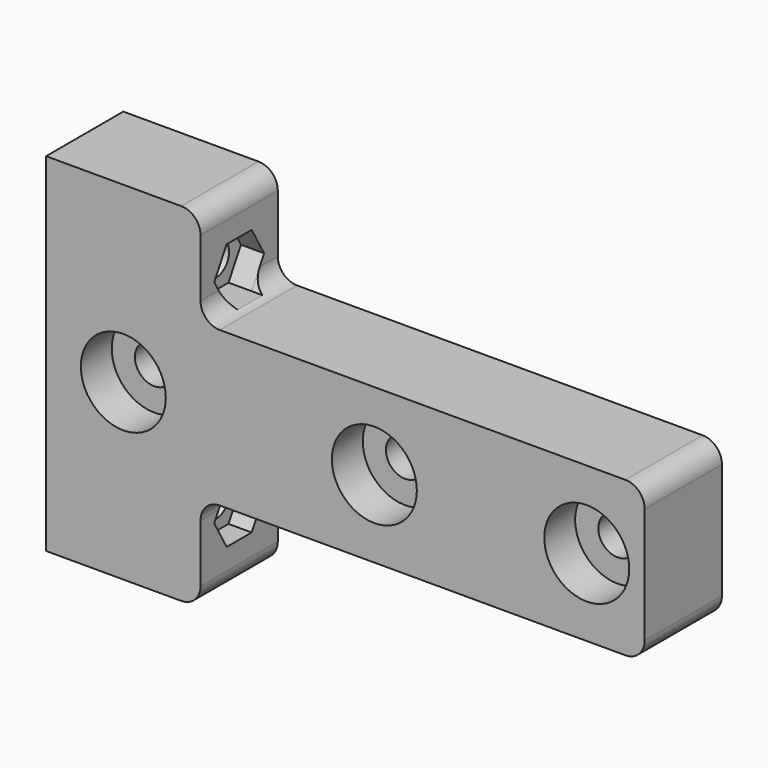
from build123d import *

# Parameters (mm, degrees)
F0_W          = 155
F0_H          = 40
F0_R          = 5
F1_DEPTH      = 25
F2_R          = 11
F3_DEPTH      = 10
F4_W          = 40
F4_H          = 25
F5_DEPTH      = 25
F6_R          = 4.25
F7_DEPTH      = 40
F9_DEPTH      = 6
F10_T4_DEPTH  = 25
F10_T10_DEPTH = 25
F10_T16_DEPTH = 25
F10_T23_DEPTH = 25
F10_T29_DEPTH = 25
F10_T35_DEPTH = 25
F10_T41_DEPTH = 25
F10_T47_DEPTH = 25
F10_T54_DEPTH = 25
F10_T60_DEPTH = 25
F10_T63_DEPTH = 50


# Not quite as in the source:
# - a fillet or chamfer that OpenCascade refuses, or shapes differently, is made with other operations: its cross-section is extruded or revolved along the edge and cut away or added


with BuildPart() as f1:
    # F0 (on Front) → F1 (new body)
    with BuildSketch(Plane.XZ):
        with Locations((-7.5, 0)):
            Rectangle(F0_W, F0_H)
        with Locations((-65, 0)):
            Circle(F0_R, mode=Mode.SUBTRACT)
        Circle(F0_R, mode=Mode.SUBTRACT)
        with Locations((55, 0)):
            Circle(F0_R, mode=Mode.SUBTRACT)
    extrude(amount=F1_DEPTH)

    # F2 (on face) → F3 (cut)
    with BuildSketch(Plane.XZ.offset(25)):
        with Locations((-65, 0)):
            Circle(F2_R)
        Circle(F2_R)
        with Locations((55, 0)):
            Circle(F2_R)
    extrude(amount=-F3_DEPTH, mode=Mode.SUBTRACT)

    # F4 (on face) → F5 (join)
    with BuildSketch(Plane(origin=(0, 0, 0), x_dir=(-1, 0, 0), z_dir=(0, 1, 0))):
        with Locations((65, 32.5)):
            Rectangle(F4_W, F4_H)
        with Locations((65, -32.5)):
            Rectangle(F4_W, F4_H)
    extrude(amount=-F5_DEPTH)

    # F6 (on face) → F7 (cut, through all)
    with BuildSketch(Plane(origin=(-85, 0, 0), x_dir=(0, -1, 0), z_dir=(-1, 0, 0))):
        with Locations((12.5, 27.5)):
            Circle(F6_R)
        with Locations((12.5, -27.5)):
            Circle(F6_R)
    extrude(amount=-F7_DEPTH, mode=Mode.SUBTRACT)

    # F8 (on face) → F9 (cut)
    with BuildSketch(Plane.YZ.offset(-45)):
        Polygon((-8.4585481157, 34.5), (-16.5414518843, 34.5), (-20.5829037687, 27.5), (-16.5414518843, 20.5), (-8.4585481157, 20.5), (-4.4170962313, 27.5), align=None)
        Polygon((-8.4585481157, -20.5), (-16.5414518843, -20.5), (-20.5829037687, -27.5), (-16.5414518843, -34.5), (-8.4585481157, -34.5), (-4.4170962313, -27.5), align=None)
    extrude(amount=-F9_DEPTH, mode=Mode.SUBTRACT)

    # F10: fillet of radius 5 on 6 edges, made by hand


with BuildPart() as f10_tool2:
    # F10_s3 → F10_t4 (new body)
    with BuildSketch(Plane.XZ):
        with BuildLine():
            ThreePointArc((-40, 20), (-43.5355339059, 21.4644660941), (-45, 25))
            Line((-45, 25), (-45, 20))
            Line((-45, 20), (-40, 20))
        make_face()
    extrude(amount=F10_T4_DEPTH)

    split(bisect_by=Plane.XY.offset(20.5), keep=Keep.BOTTOM)

    split(bisect_by=Plane(origin=(0, -15.2206714755, 8.7876587737), x_dir=(1, 0, 0), z_dir=(0, 0.8660254038, -0.5)), keep=Keep.TOP)


with BuildPart() as f1_1:
    add(f1.part)

    # F10_t1: union F10_tool2
    add(f10_tool2.part)


with BuildPart() as f10_tool8:
    # F10_s9 → F10_t10 (new body)
    with BuildSketch(Plane.XZ):
        with BuildLine():
            ThreePointArc((-40, 20), (-43.5355339059, 21.4644660941), (-45, 25))
            Line((-45, 25), (-45, 20))
            Line((-45, 20), (-40, 20))
        make_face()
    extrude(amount=F10_T10_DEPTH)

    split(bisect_by=Plane.XY.offset(20.5), keep=Keep.TOP)

    split(bisect_by=Plane(origin=(0, -15.2206714755, 8.7876587737), x_dir=(1, 0, 0), z_dir=(0, 0.8660254038, -0.5)), keep=Keep.TOP)


with BuildPart() as f1_2:
    add(f1_1.part)

    # F10_t7: union F10_tool8
    add(f10_tool8.part)


with BuildPart() as f10_tool14:
    # F10_s15 → F10_t16 (new body)
    with BuildSketch(Plane.XZ):
        with BuildLine():
            ThreePointArc((-40, 20), (-43.5355339059, 21.4644660941), (-45, 25))
            Line((-45, 25), (-45, 20))
            Line((-45, 20), (-40, 20))
        make_face()
    extrude(amount=F10_T16_DEPTH)

    split(bisect_by=Plane(origin=(0, -3.5293285245, -2.0376587737), x_dir=(1, 0, 0), z_dir=(0, 0.8660254038, 0.5)), keep=Keep.TOP)

    split(bisect_by=Plane.XY.offset(20.5), keep=Keep.BOTTOM)

    split(bisect_by=Plane(origin=(0, -15.2206714755, 8.7876587737), x_dir=(1, 0, 0), z_dir=(0, -0.8660254038, 0.5)), keep=Keep.TOP)


with BuildPart() as f1_3:
    add(f1_2.part)

    # F10_t13: union F10_tool14
    add(f10_tool14.part)


with BuildPart() as f10_tool21:
    # F10_s22 → F10_t23 (new body)
    with BuildSketch(Plane.XZ):
        with BuildLine():
            ThreePointArc((-40, 20), (-43.5355339059, 21.4644660941), (-45, 25))
            Line((-45, 25), (-45, 20))
            Line((-45, 20), (-40, 20))
        make_face()
    extrude(amount=F10_T23_DEPTH)

    split(bisect_by=Plane(origin=(0, -3.5293285245, -2.0376587737), x_dir=(1, 0, 0), z_dir=(0, -0.8660254038, -0.5)), keep=Keep.TOP)

    split(bisect_by=Plane.XY.offset(20.5), keep=Keep.BOTTOM)


with BuildPart() as f1_4:
    add(f1_3.part)

    # F10_t20: union F10_tool21
    add(f10_tool21.part)


with BuildPart() as f10_tool27:
    # F10_s28 → F10_t29 (new body)
    with BuildSketch(Plane.XZ):
        with BuildLine():
            ThreePointArc((-40, 20), (-43.5355339059, 21.4644660941), (-45, 25))
            Line((-45, 25), (-45, 20))
            Line((-45, 20), (-40, 20))
        make_face()
    extrude(amount=F10_T29_DEPTH)

    split(bisect_by=Plane(origin=(0, -3.5293285245, -2.0376587737), x_dir=(1, 0, 0), z_dir=(0, -0.8660254038, -0.5)), keep=Keep.TOP)

    split(bisect_by=Plane.XY.offset(20.5), keep=Keep.TOP)


with BuildPart() as f1_5:
    add(f1_4.part)

    # F10_t26: union F10_tool27
    add(f10_tool27.part)


with BuildPart() as f10_tool33:
    # F10_s34 → F10_t35 (new body)
    with BuildSketch(Plane.XZ):
        with BuildLine():
            ThreePointArc((-40, -20), (-43.5355339059, -21.4644660941), (-45, -25))
            Line((-45, -25), (-45, -20))
            Line((-45, -20), (-40, -20))
        make_face()
    extrude(amount=F10_T35_DEPTH)

    split(bisect_by=Plane.XY.offset(-20.5), keep=Keep.TOP)

    split(bisect_by=Plane(origin=(0, -15.2206714755, -8.7876587737), x_dir=(1, 0, 0), z_dir=(0, 0.8660254038, 0.5)), keep=Keep.TOP)


with BuildPart() as f1_6:
    add(f1_5.part)

    # F10_t32: union F10_tool33
    add(f10_tool33.part)


with BuildPart() as f10_tool39:
    # F10_s40 → F10_t41 (new body)
    with BuildSketch(Plane.XZ):
        with BuildLine():
            ThreePointArc((-40, -20), (-43.5355339059, -21.4644660941), (-45, -25))
            Line((-45, -25), (-45, -20))
            Line((-45, -20), (-40, -20))
        make_face()
    extrude(amount=F10_T41_DEPTH)

    split(bisect_by=Plane.XY.offset(-20.5), keep=Keep.BOTTOM)

    split(bisect_by=Plane(origin=(0, -15.2206714755, -8.7876587737), x_dir=(1, 0, 0), z_dir=(0, 0.8660254038, 0.5)), keep=Keep.TOP)


with BuildPart() as f1_7:
    add(f1_6.part)

    # F10_t38: union F10_tool39
    add(f10_tool39.part)


with BuildPart() as f10_tool45:
    # F10_s46 → F10_t47 (new body)
    with BuildSketch(Plane.XZ):
        with BuildLine():
            ThreePointArc((-40, -20), (-43.5355339059, -21.4644660941), (-45, -25))
            Line((-45, -25), (-45, -20))
            Line((-45, -20), (-40, -20))
        make_face()
    extrude(amount=F10_T47_DEPTH)

    split(bisect_by=Plane.XY.offset(-20.5), keep=Keep.TOP)

    split(bisect_by=Plane(origin=(0, -3.5293285245, 2.0376587737), x_dir=(1, 0, 0), z_dir=(0, 0.8660254038, -0.5)), keep=Keep.TOP)

    split(bisect_by=Plane(origin=(0, -15.2206714755, -8.7876587737), x_dir=(1, 0, 0), z_dir=(0, -0.8660254038, -0.5)), keep=Keep.TOP)


with BuildPart() as f1_8:
    add(f1_7.part)

    # F10_t44: union F10_tool45
    add(f10_tool45.part)


with BuildPart() as f10_tool52:
    # F10_s53 → F10_t54 (new body)
    with BuildSketch(Plane.XZ):
        with BuildLine():
            ThreePointArc((-40, -20), (-43.5355339059, -21.4644660941), (-45, -25))
            Line((-45, -25), (-45, -20))
            Line((-45, -20), (-40, -20))
        make_face()
    extrude(amount=F10_T54_DEPTH)

    split(bisect_by=Plane.XY.offset(-20.5), keep=Keep.TOP)

    split(bisect_by=Plane(origin=(0, -3.5293285245, 2.0376587737), x_dir=(1, 0, 0), z_dir=(0, -0.8660254038, 0.5)), keep=Keep.TOP)


with BuildPart() as f1_9:
    add(f1_8.part)

    # F10_t51: union F10_tool52
    add(f10_tool52.part)


with BuildPart() as f10_tool58:
    # F10_s59 → F10_t60 (new body)
    with BuildSketch(Plane.XZ):
        with BuildLine():
            ThreePointArc((-40, -20), (-43.5355339059, -21.4644660941), (-45, -25))
            Line((-45, -25), (-45, -20))
            Line((-45, -20), (-40, -20))
        make_face()
    extrude(amount=F10_T60_DEPTH)

    split(bisect_by=Plane.XY.offset(-20.5), keep=Keep.BOTTOM)

    split(bisect_by=Plane(origin=(0, -3.5293285245, 2.0376587737), x_dir=(1, 0, 0), z_dir=(0, -0.8660254038, 0.5)), keep=Keep.TOP)


with BuildPart() as f1_10:
    add(f1_9.part)

    # F10_t57: union F10_tool58
    add(f10_tool58.part)

    # F10_s64 → F10_t63 (cut)
    with BuildSketch(Plane.XZ.offset(-12.5)):
        with BuildLine():
            ThreePointArc((-50, 45), (-46.4644660941, 43.5355339059), (-45, 40))
            Line((-45, 40), (-45, 45))
            Line((-45, 45), (-50, 45))
        make_face()
        with BuildLine():
            ThreePointArc((-45, -40), (-46.4644660941, -43.5355339059), (-50, -45))
            Line((-50, -45), (-45, -45))
            Line((-45, -45), (-45, -40))
        make_face()
        with BuildLine():
            ThreePointArc((70, -15), (68.5355339059, -18.5355339059), (65, -20))
            Line((65, -20), (70, -20))
            Line((70, -20), (70, -15))
        make_face()
        with BuildLine():
            ThreePointArc((70, 15), (68.5355339059, 18.5355339059), (65, 20))
            Line((65, 20), (70, 20))
            Line((70, 20), (70, 15))
        make_face()
    extrude(amount=F10_T63_DEPTH, mode=Mode.SUBTRACT)


solid = f1_10.part
